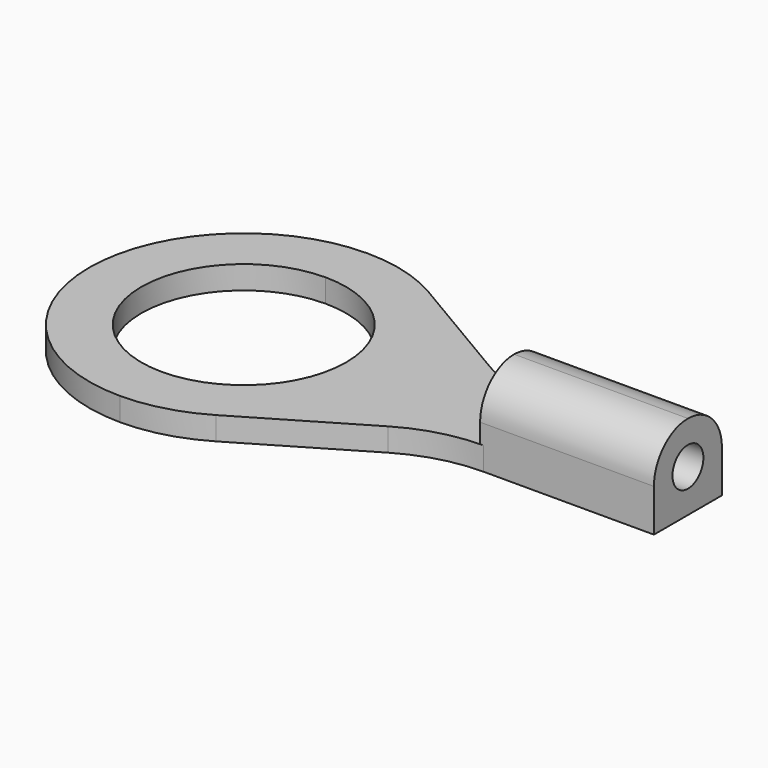
from build123d import *

# Parameters (mm, degrees)
F1_DEPTH = 0.6
F2_W     = 4.5
F2_H     = 2.2
F3_DEPTH = 1.6
F4_R     = 1.09999
F5_R     = 0.5
F6_DEPTH = 25


# Not quite as in the source:
# - a fillet or chamfer is up to 0.001 mm smaller than in the source, because OpenCascade refuses the exact size


with BuildPart() as f1:
    # F0 (on Top) → F1 (new body)
    with BuildSketch(Plane.XY):
        with BuildLine():
            Line((11.0937791562, 2.9), (15.5, 2.9))
            Line((15.5, 2.9), (15.5, 5.1))
            Line((15.5, 5.1), (11.0937791562, 5.1))
            ThreePointArc((11.0937791562, 5.1), (10.0387329979, 5.2416483307), (9.0584096032, 5.656561198))
            Line((9.0584096032, 5.656561198), (6.035369553, 7.443438802))
            ThreePointArc((6.035369553, 7.443438802), (5.0550461583, 7.8583516693), (4, 8))
            Line((4, 8), (4, 6.65))
            ThreePointArc((4, 6.65), (5.8738329701, 5.8738329701), (6.65, 4))
            ThreePointArc((6.65, 4), (5.8738329701, 2.1261670299), (4, 1.35))
            Line((4, 1.35), (4, 0))
            ThreePointArc((4, 0), (5.0550461583, 0.1416483307), (6.035369553, 0.556561198))
            Line((6.035369553, 0.556561198), (9.0584096032, 2.343438802))
            ThreePointArc((9.0584096032, 2.343438802), (10.0387329979, 2.7583516693), (11.0937791562, 2.9))
        make_face()
        with BuildLine():
            ThreePointArc((0, 4), (1.1715728753, 1.1715728753), (4, 0))
            Line((4, 0), (4, 1.35))
            ThreePointArc((4, 1.35), (1.35, 4), (4, 6.65))
            Line((4, 6.65), (4, 8))
            ThreePointArc((4, 8), (1.1715728753, 6.8284271247), (0, 4))
        make_face()
    extrude(amount=F1_DEPTH)

    # F2 (on face) → F3 (join)
    with BuildSketch(Plane.XY.offset(0.6)):
        with Locations((13.25, 4)):
            Rectangle(F2_W, F2_H)
    extrude(amount=F3_DEPTH)

    # F4 (radius 1.1 in the source; OpenCascade refuses exactly that, so slightly less here)
    f4_edges = [f1.edges().sort_by_distance(p)[0] for p in [
        (13.25, 5.1, 2.2),
        (13.25, 2.9, 2.2),
    ]]
    fillet(f4_edges, radius=F4_R)

    # F5 (on face) → F6 (cut)
    with BuildSketch(Plane.YZ.offset(15.5)):
        with Locations((4, 1.1)):
            Circle(F5_R)
    extrude(amount=-F6_DEPTH, mode=Mode.SUBTRACT)


solid = f1.part
